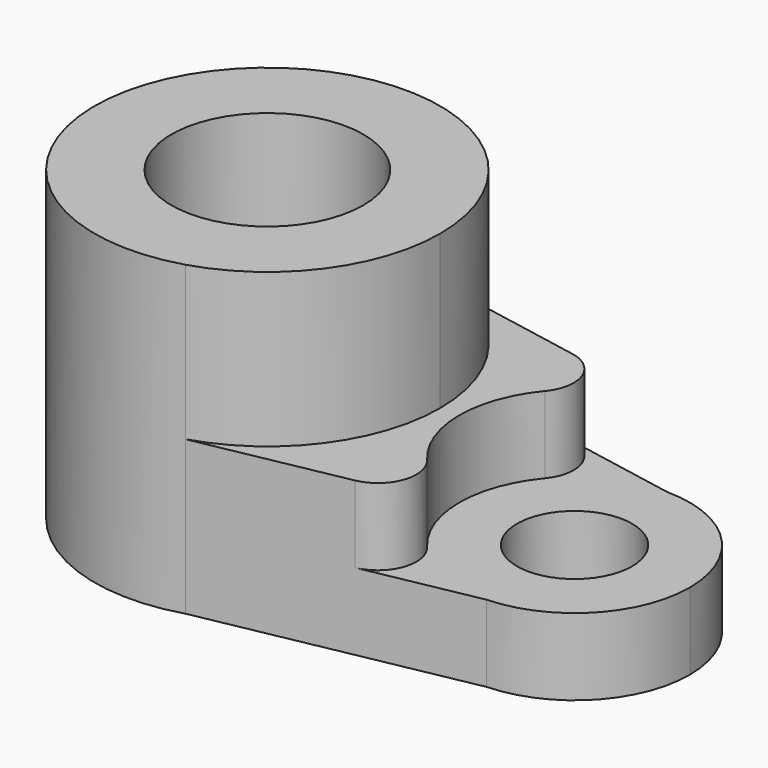
from build123d import *

# Parameters (mm, degrees)
F0_R     = 15.875
F0_R_2   = 9.525
F1_DEPTH = 25.4
F2_DEPTH = 25.4
F3_DEPTH = 12.7
F4_R     = 6.35


with BuildPart() as f1:
    # F0 (on Top) → F1 (new body)
    with BuildSketch(Plane.XY):
        with BuildLine():
            ThreePointArc((8.2981181618, -27.3435890105), (22.9526616264, -17.0207505493), (28.575, 0))
            ThreePointArc((28.575, 0), (23.5615881585, 16.16731853), (10.2805336167, 26.6616063574))
            ThreePointArc((10.2805336167, 26.6616063574), (-28.5557674937, 1.0482212761), (8.2981181618, -27.3435890105))
        make_face()
        Circle(F0_R, mode=Mode.SUBTRACT)
        with BuildLine():
            ThreePointArc((69.85, 0), (64.2983142533, 13.442396078), (50.8790800715, 19.0498358613))
            ThreePointArc((50.8790800715, 19.0498358613), (31.7523183533, -0.2971933484), (51.4733508184, -19.0380959835))
            ThreePointArc((51.4733508184, -19.0380959835), (64.5063823289, -13.2301770001), (69.85, 0))
        make_face()
        with Locations((50.8, 0)):
            Circle(F0_R_2, mode=Mode.SUBTRACT)
        with BuildLine():
            ThreePointArc((10.2805336167, 26.6616063574), (23.5615881585, 16.16731853), (28.575, 0))
            ThreePointArc((28.575, 0), (22.9526616264, -17.0207505493), (8.2981181618, -27.3435890105))
            Line((8.2981181618, -27.3435890105), (51.4733508184, -19.0380959835))
            ThreePointArc((51.4733508184, -19.0380959835), (31.7523183533, -0.2971933484), (50.8790800715, 19.0498358613))
            Line((50.8790800715, 19.0498358613), (10.2805336167, 26.6616063574))
        make_face()
    extrude(amount=-F1_DEPTH)

    # F0 (on Top) → F2 (join)
    with BuildSketch(Plane.XY):
        with BuildLine():
            ThreePointArc((8.2981181618, -27.3435890105), (22.9526616264, -17.0207505493), (28.575, 0))
            ThreePointArc((28.575, 0), (23.5615881585, 16.16731853), (10.2805336167, 26.6616063574))
            ThreePointArc((10.2805336167, 26.6616063574), (-28.5557674937, 1.0482212761), (8.2981181618, -27.3435890105))
        make_face()
        Circle(F0_R, mode=Mode.SUBTRACT)
    extrude(amount=F2_DEPTH)

    # F0 (on Top) → F3 (cut)
    with BuildSketch(Plane.XY):
        with BuildLine():
            ThreePointArc((69.85, 0), (64.2983142533, 13.442396078), (50.8790800715, 19.0498358613))
            ThreePointArc((50.8790800715, 19.0498358613), (31.7523183533, -0.2971933484), (51.4733508184, -19.0380959835))
            ThreePointArc((51.4733508184, -19.0380959835), (64.5063823289, -13.2301770001), (69.85, 0))
        make_face()
        with Locations((50.8, 0)):
            Circle(F0_R_2, mode=Mode.SUBTRACT)
    extrude(amount=-F3_DEPTH, mode=Mode.SUBTRACT)

    # F4
    f4_edges = [f1.edges().sort_by_distance(p)[0] for p in [
        (51.473351, -19.038096, -6.35),
        (50.87908, 19.049836, -6.35),
    ]]
    fillet(f4_edges, radius=F4_R)


solid = f1.part
